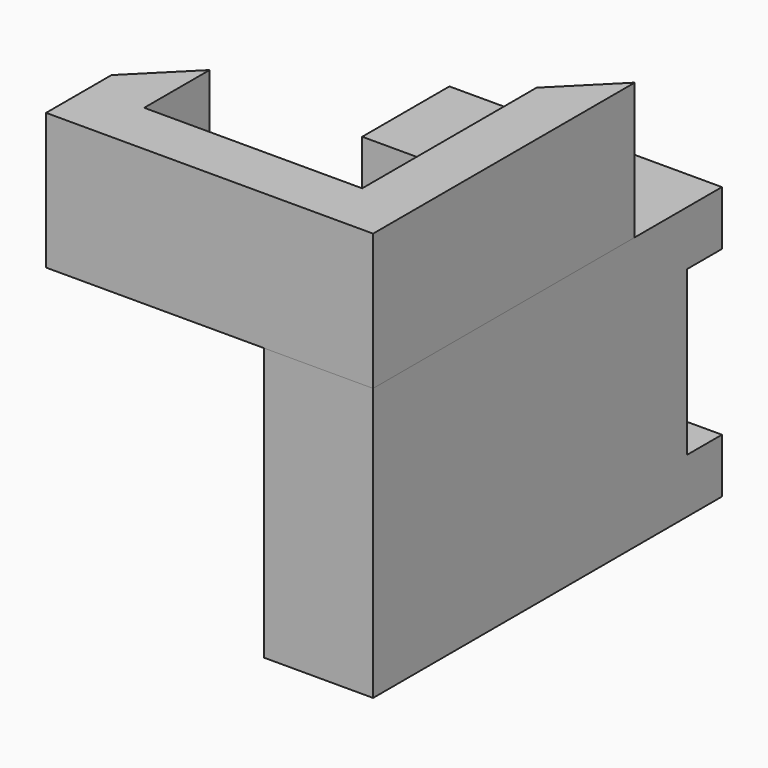
from build123d import *

# Parameters (mm, degrees)
F1_DEPTH = 25
F2_W     = 60
F2_H     = 50
F3_DEPTH = 20
F4_DEPTH = 50


with BuildPart() as f1:
    # F0 (on Top) → F1 (new body)
    with BuildSketch(Plane.XY):
        Polygon((-60, -45), (-60, -60), (0, -60), (0, 0), (-10, -10), (-10, -50), (-50, -50), (-50, -35), align=None)
    extrude(amount=F1_DEPTH)


with BuildPart() as f3:
    # F2 (on Right) → F3 (new body)
    with BuildSketch(Plane.YZ):
        with Locations((-30, -25)):
            Rectangle(F2_W, F2_H)
    extrude(amount=-F3_DEPTH)

    # F2 (on Right) → F4 (join)
    with BuildSketch(Plane.YZ):
        Polygon((0, 0), (0, -50), (20, -50), (20, -40), (12, -40), (12, -10), (20, -10), (20, 0), align=None)
    extrude(amount=-F4_DEPTH)


solid = Compound([f1.part, f3.part])
